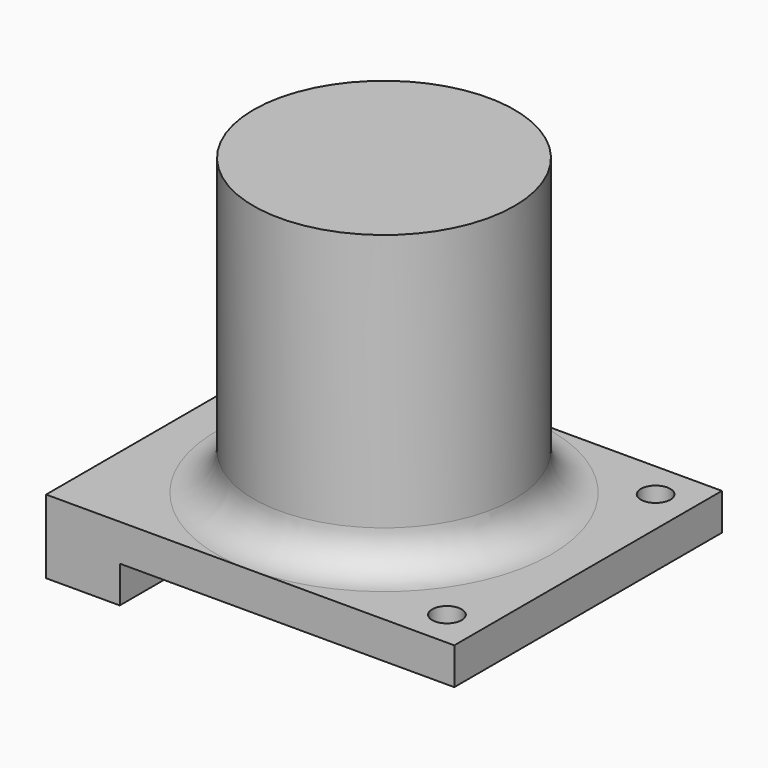
from build123d import *

# Parameters (mm, degrees)
F0_R     = 2
F1_DEPTH = 5
F2_DEPTH = 45
F3_DEPTH = 5
F4_DEPTH = 5
F5_R     = 4.99999


# Not quite as in the source:
# - a fillet or chamfer is up to 0.001 mm smaller than in the source, because OpenCascade refuses the exact size


with BuildPart() as f1:
    # F0 (on Top) → F1 (new body)
    with BuildSketch(Plane.XY):
        Polygon((-17.7, 22.7), (-17.7, 0), (-17.7, -22.7), (27.7, -22.7), (27.7, 22.7), align=None)
        with Locations((22.7, -17.7)):
            Circle(F0_R, mode=Mode.SUBTRACT)
        with BuildLine():
            ThreePointArc((-17.7, 0), (0, 17.7), (17.7, 0))
            ThreePointArc((17.7, 0), (0, -17.7), (-17.7, 0))
        make_face(mode=Mode.SUBTRACT)
        with Locations((22.7, 17.7)):
            Circle(F0_R, mode=Mode.SUBTRACT)
        with BuildLine():
            ThreePointArc((-17.7, 0), (0, -17.7), (17.7, 0))
            ThreePointArc((17.7, 0), (0, 17.7), (-17.7, 0))
        make_face()
    extrude(amount=F1_DEPTH)

    # F0 (on Top) → F2 (join)
    with BuildSketch(Plane.XY):
        with BuildLine():
            ThreePointArc((-17.7, 0), (0, -17.7), (17.7, 0))
            ThreePointArc((17.7, 0), (0, 17.7), (-17.7, 0))
        make_face()
    extrude(amount=F2_DEPTH)

    # F0 (on Top) → F3 (join, through all)
    with BuildSketch(Plane.XY):
        Polygon((-17.7, -22.7), (-17.7, 0), (-17.7, 22.7), (-27.7, 22.7), (-27.7, -22.7), align=None)
    extrude(amount=F3_DEPTH)

    # F0 (on Top) → F4 (join)
    with BuildSketch(Plane.XY):
        Polygon((-17.7, -22.7), (-17.7, 0), (-17.7, 22.7), (-27.7, 22.7), (-27.7, -22.7), align=None)
    extrude(amount=-F4_DEPTH)

    # F5 (radius 5 in the source; OpenCascade refuses exactly that, so slightly less here)
    f5_edges = [f1.edges().sort_by_distance(p)[0] for p in [
        (-17.7, 0, 5),
    ]]
    fillet(f5_edges, radius=F5_R)


solid = f1.part
